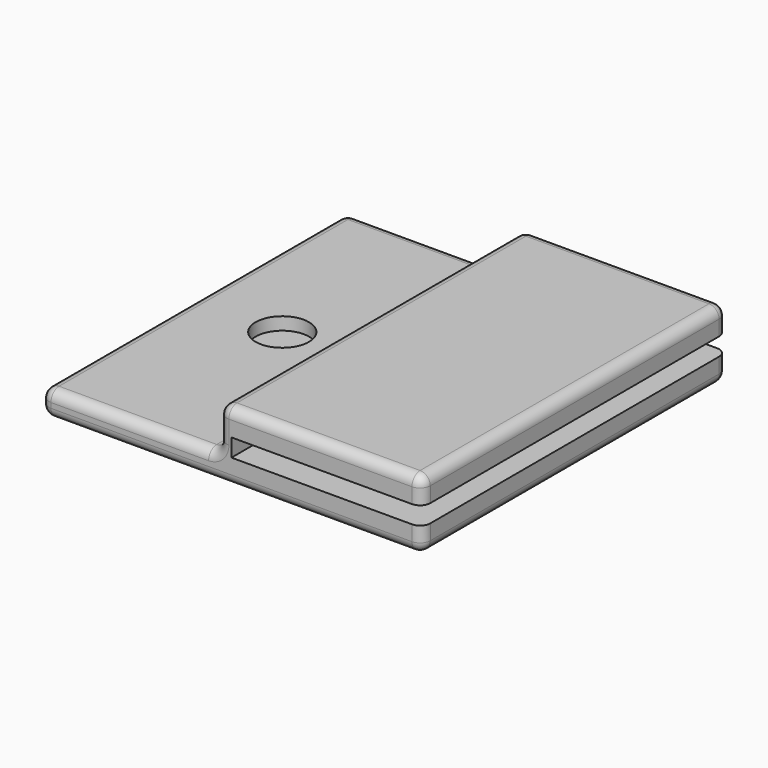
from build123d import *

# Parameters (mm, degrees)
F0_W     = 75
F0_H     = 75
F1_DEPTH = 5
F2_W     = 40
F2_H     = 75
F3_DEPTH = 8.5
F4_W     = 75
F4_H     = 3.5
F5_DEPTH = 37.5
F6_R     = 5.25
F7_DEPTH = 2.5
F8_R     = 2


with BuildPart() as f1:
    # F0 (on Top) → F1 (new body)
    with BuildSketch(Plane.XY):
        Rectangle(F0_W, F0_H)
    extrude(amount=F1_DEPTH)

    # F2 (on face) → F3 (join)
    with BuildSketch(Plane.XY.offset(5)):
        with Locations((17.5, 0)):
            Rectangle(F2_W, F2_H)
    extrude(amount=F3_DEPTH)

    # F4 (on face) → F5 (cut, through all)
    with BuildSketch(Plane.YZ.offset(37.5)):
        with Locations((0, 6.75)):
            Rectangle(F4_W, F4_H)
    extrude(amount=-F5_DEPTH, mode=Mode.SUBTRACT)

    # F6 (on face) → F7 (cut)
    with BuildSketch(Plane.XY.offset(5)):
        with Locations((-20, 0)):
            Circle(F6_R)
    extrude(amount=-F7_DEPTH, mode=Mode.SUBTRACT)

    # F8
    f8_edges = [f1.edges().sort_by_distance(p)[0] for p in [
        (17.5, 37.5, 13.5),
        (-2.5, 0, 13.5),
        (17.5, -37.5, 13.5),
        (37.5, 0, 13.5),
        (-2.5, 37.5, 9.25),
        (-2.5, -37.5, 9.25),
        (-2.5, 0, 5),
        (-37.5, 37.5, 2.5),
        (-37.5, -37.5, 2.5),
        (-37.5, 0, 0),
        (-37.5, 0, 5),
        (0, -37.5, 0),
        (37.5, 0, 0),
        (0, 37.5, 0),
        (37.5, -37.5, 11),
        (37.5, -37.5, 2.5),
        (37.5, 37.5, 11),
        (37.5, 37.5, 2.5),
        (-20, -37.5, 5),
        (-20, 37.5, 5),
    ]]
    fillet(f8_edges, radius=F8_R)


solid = f1.part
